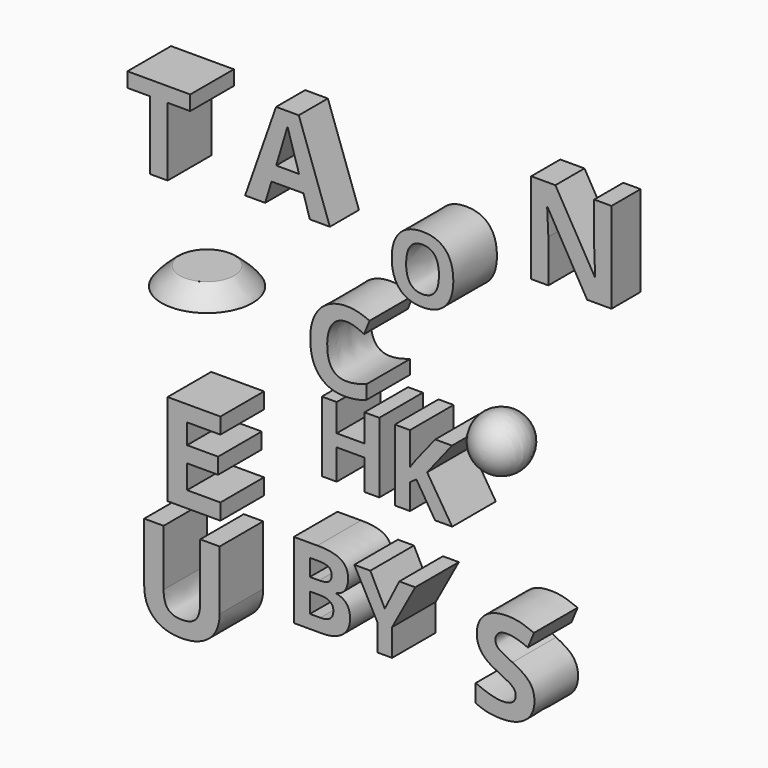
from build123d import *

# Parameters (mm, degrees)
F0_TEXT_SIZE  = 29.9906279288
F1_DEPTH      = 15
F2_R          = 12.5
F3_DEPTH      = 5
F7_TEXT_SIZE  = 27.0384452894
F8_DEPTH      = 15
F9_TEXT_SIZE  = 35.349351008
F10_DEPTH     = 15
F11_TEXT_SIZE = 34.7165717385
F12_DEPTH     = 15
F13_TEXT_SIZE = 29.2370945637
F14_DEPTH     = 15
F15_TEXT_SIZE = 24.9172668873
F16_DEPTH     = 15
F17_TEXT_SIZE = 32.0560981718
F18_DEPTH     = 15
F19_TEXT_SIZE = 33.8018250962
F20_DEPTH     = 10
F21_TEXT_SIZE = 34.901070305
F22_DEPTH     = 10
F23_TEXT_SIZE = 27.4811557675
F24_DEPTH     = 15
F25_TEXT_SIZE = 26.8638806625
F26_DEPTH     = 15
F27_TEXT_SIZE = 35.410364055
F28_DEPTH     = 15


# Not quite as in the source:
# - a fillet or chamfer that OpenCascade refuses, or shapes differently, is made with other operations: its cross-section is extruded or revolved along the edge and cut away or added
# - Text() gives the source's letters only with a copy of the font that has no kerning and outlines rounded to 1/6400 em; it was checked with that copy


with BuildPart() as f1:
    # F0 (on Front) → F1 (new body)
    with BuildSketch(Plane.XZ):
        with Locations((-10, 0)):
            Text('C', F0_TEXT_SIZE, font='Open Sans', font_style=FontStyle.BOLD, text_align=(TextAlign.LEFT, TextAlign.BOTTOM))
    extrude(amount=F1_DEPTH)


with BuildPart() as f3:
    # F2 (on Top) → F3 (new body)
    with BuildSketch(Plane.XY):
        with Locations((-53.4992665052, 6.0633448884)):
            Circle(F2_R)
    extrude(amount=F3_DEPTH)

    # F4: fillet of radius 5 on 1 edges, made by hand

    # F4_s1 → F4_t2 (revolve, cut)
    with BuildSketch(Plane.XZ.offset(-6.0633448884)):
        with BuildLine():
            add(Edge.make_bspline(
                [(-40.9992665052, 0), (-40.9992665052, 5), (-45.9992665052, 5)],
                knots=[0, 0, 0, 1, 1, 1], degree=2, weights=[1, 0.1111111111, 1]))
            Line((-45.9992665052, 5), (-40.9992665052, 5))
            Line((-40.9992665052, 5), (-40.9992665052, 0))
        make_face()
    revolve(axis=Axis((-53.4992665052, 6.0633448884, 5), (0, 0, 1)), mode=Mode.SUBTRACT)


with BuildPart() as f6:
    # F5 (on Top) → F6 (revolve)
    with BuildSketch(Plane.XY):
        with BuildLine():
            Line((40.9858538571, -18.2743860581), (40.9858538571, -3.2744047977))
            ThreePointArc((40.9858538571, -3.2744047977), (33.4739986062, -10.7743954279), (40.9858538571, -18.2743860581))
        make_face()
    revolve(axis=Axis((40.9858538571, -10.7743954279, 0), (0, -1, 0)))


with BuildPart() as f8:
    # F7 (on Front) → F8 (new body)
    with BuildSketch(Plane.XZ):
        with Locations((-7.4950577362, -21.7064645945)):
            Text('H', F7_TEXT_SIZE, font='Open Sans', font_style=FontStyle.BOLD, text_align=(TextAlign.LEFT, TextAlign.BOTTOM))
    extrude(amount=F8_DEPTH)


with BuildPart() as f10:
    # F9 (on Front) → F10 (new body)
    with BuildSketch(Plane.XZ):
        with Locations((-50.6826529283, -41.558353087)):
            Text('E', F9_TEXT_SIZE, font='Open Sans', font_style=FontStyle.BOLD, text_align=(TextAlign.LEFT, TextAlign.BOTTOM))
    extrude(amount=F10_DEPTH)


with BuildPart() as f12:
    # F11 (on Front) → F12 (new body)
    with BuildSketch(Plane.XZ):
        with Locations((35.6946838193, -64.0571644284)):
            Text('S', F11_TEXT_SIZE, font='Open Sans', font_style=FontStyle.BOLD, text_align=(TextAlign.LEFT, TextAlign.BOTTOM))
    extrude(amount=F12_DEPTH)


with BuildPart() as f14:
    # F13 (on Front) → F14 (new body)
    with BuildSketch(Plane.XZ):
        with Locations((-15.3993622572, -59.7786111148)):
            Text('B', F13_TEXT_SIZE, font='Open Sans', font_style=FontStyle.BOLD, text_align=(TextAlign.LEFT, TextAlign.BOTTOM))
    extrude(amount=F14_DEPTH)


with BuildPart() as f16:
    # F15 (on Front) → F16 (new body)
    with BuildSketch(Plane.XZ):
        with Locations((12.7297645057, 28.4858894888)):
            Text('O', F15_TEXT_SIZE, font='Open Sans', font_style=FontStyle.BOLD, text_align=(TextAlign.LEFT, TextAlign.BOTTOM))
    extrude(amount=F16_DEPTH)


with BuildPart() as f18:
    # F17 (on Front) → F18 (new body)
    with BuildSketch(Plane.XZ):
        with Locations((-59.1997031663, 36.1193124826)):
            Text('T', F17_TEXT_SIZE, font='Open Sans', font_style=FontStyle.BOLD, text_align=(TextAlign.LEFT, TextAlign.BOTTOM))
    extrude(amount=F18_DEPTH)


with BuildPart() as f20:
    # F19 (on Front) → F20 (new body)
    with BuildSketch(Plane.XZ):
        with Locations((-30.1743112504, 36.1102409661)):
            Text('A', F19_TEXT_SIZE, font='Open Sans', font_style=FontStyle.BOLD, text_align=(TextAlign.LEFT, TextAlign.BOTTOM))
    extrude(amount=F20_DEPTH)


with BuildPart() as f22:
    # F21 (on Front) → F22 (new body)
    with BuildSketch(Plane.XZ):
        with Locations((45.4098619521, 41.452575475)):
            Text('N', F21_TEXT_SIZE, font='Open Sans', font_style=FontStyle.BOLD, text_align=(TextAlign.LEFT, TextAlign.BOTTOM))
    extrude(amount=F22_DEPTH)


with BuildPart() as f24:
    # F23 (on Front) → F24 (new body)
    with BuildSketch(Plane.XZ):
        with Locations((12.5643843785, -22.2597364336)):
            Text('K', F23_TEXT_SIZE, font='Open Sans', font_style=FontStyle.BOLD, text_align=(TextAlign.LEFT, TextAlign.BOTTOM))
    extrude(amount=F24_DEPTH)


with BuildPart() as f26:
    # F25 (on Front) → F26 (new body)
    with BuildSketch(Plane.XZ):
        with Locations((3.8734450936, -59.4260282815)):
            Text('Y', F25_TEXT_SIZE, font='Open Sans', font_style=FontStyle.BOLD, text_align=(TextAlign.LEFT, TextAlign.BOTTOM))
    extrude(amount=F26_DEPTH)


with BuildPart() as f28:
    # F27 (on Front) → F28 (new body)
    with BuildSketch(Plane.XZ):
        with Locations((-56.9478087127, -73.1505304575)):
            Text('U', F27_TEXT_SIZE, font='Open Sans', font_style=FontStyle.BOLD, text_align=(TextAlign.LEFT, TextAlign.BOTTOM))
    extrude(amount=F28_DEPTH)


solid = Compound([f1.part, f3.part, f6.part, f8.part, f10.part, f12.part, f14.part, f16.part, f18.part, f20.part, f22.part, f24.part, f26.part, f28.part])
